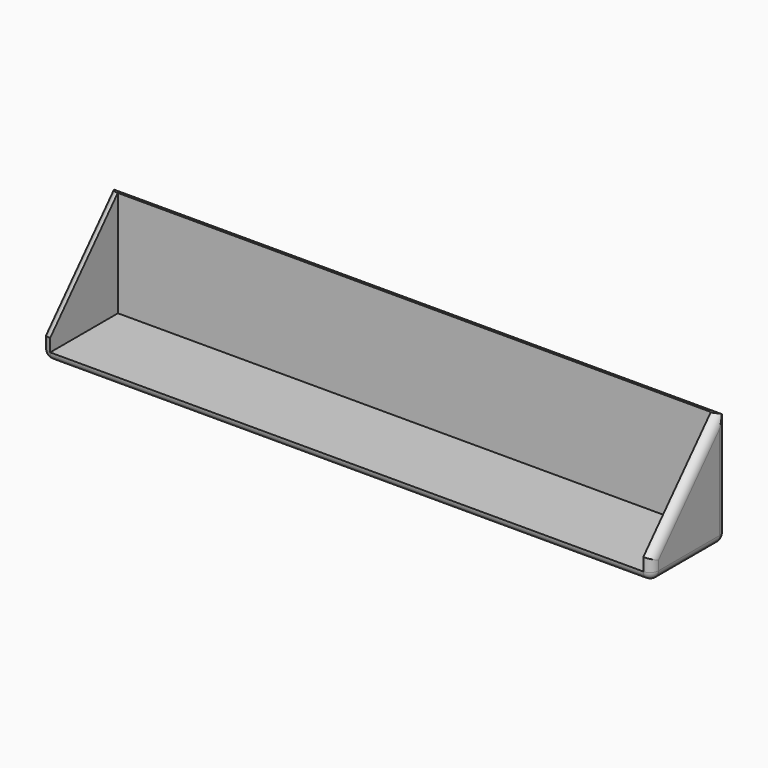
from build123d import *

# Parameters (mm, degrees)
F0_W         = 144
F0_H         = 22
F1_DEPTH     = 2
F3_DEPTH     = 25
F5_DEPTH     = 160
F6_T1_DEPTH  = 18
F6_T3_DEPTH  = 140
F6_T5_DEPTH  = 30
F6_T7_DEPTH  = 39.6649624979
F6_T9_DEPTH  = 8
F6_T11_DEPTH = 154
F6_S15_W     = 2
F6_S15_H     = 2
F6_T16_DEPTH = 2
F6_S21_W     = 2
F6_S21_H     = 2
F6_T22_DEPTH = 2
F6_S27_W     = 2
F6_S27_H     = 2
F6_T28_DEPTH = 2
F6_S33_W     = 2
F6_S33_H     = 2
F6_T34_DEPTH = 2


# Not quite as in the source:
# - a fillet or chamfer that OpenCascade refuses, or shapes differently, is made with other operations: its cross-section is extruded or revolved along the edge and cut away or added


with BuildPart() as f1:
    # F0 (on Top) → F1 (new body)
    with BuildSketch(Plane.XY):
        Rectangle(F0_W, F0_H)
    extrude(amount=F1_DEPTH)

    # F2 (on face) → F3 (join)
    with BuildSketch(Plane.XY.offset(2)):
        Polygon((-70.000000298, -11), (-70.000000298, 9.000000298), (70.000000298, 9.000000298), (70.000000298, -11), (72, -11), (72, 11), (-72, 11), (-72, -11), align=None)
    extrude(amount=F3_DEPTH)

    # F4 (on face) → F5 (cut)
    with BuildSketch(Plane(origin=(-72, 0, 0), x_dir=(0, -1, 0), z_dir=(-1, 0, 0))):
        Polygon((11, 27), (-8.9, 27), (11, 5), align=None)
    extrude(amount=-F5_DEPTH, mode=Mode.SUBTRACT)

    # F6: fillet of radius 2 on 11 edges, made by hand

    # F6_s2 → F6_t1 (cut)
    with BuildSketch(Plane.XZ.offset(-9)):
        with BuildLine():
            ThreePointArc((72, 2), (71.4142135624, 0.5857864376), (70, 0))
            Line((70, 0), (72, 0))
            Line((72, 0), (72, 2))
        make_face()
        with BuildLine():
            ThreePointArc((-70, 0), (-71.4142135624, 0.5857864376), (-72, 2))
            Line((-72, 2), (-72, 0))
            Line((-72, 0), (-70, 0))
        make_face()
    extrude(amount=F6_T1_DEPTH, mode=Mode.SUBTRACT)

    # F6_s4 → F6_t3 (cut)
    with BuildSketch(Plane.YZ.offset(-70)):
        with BuildLine():
            ThreePointArc((9, 0), (10.4142135624, 0.5857864376), (11, 2))
            Line((11, 2), (11, 0))
            Line((11, 0), (9, 0))
        make_face()
        with BuildLine():
            ThreePointArc((-11, 2), (-10.4142135624, 0.5857864376), (-9, 0))
            Line((-9, 0), (-11, 0))
            Line((-11, 0), (-11, 2))
        make_face()
    extrude(amount=F6_T3_DEPTH, mode=Mode.SUBTRACT)

    # F6_s6 → F6_t5 (cut)
    with BuildSketch(Plane.XY.offset(2)):
        with BuildLine():
            ThreePointArc((-70, 11), (-71.4142135624, 10.4142135624), (-72, 9))
            Line((-72, 9), (-72, 11))
            Line((-72, 11), (-70, 11))
        make_face()
        with BuildLine():
            ThreePointArc((72, 9), (71.4142135624, 10.4142135624), (70, 11))
            Line((70, 11), (72, 11))
            Line((72, 11), (72, 9))
        make_face()
    extrude(amount=F6_T5_DEPTH, mode=Mode.SUBTRACT)

    # F6_s8 → F6_t7 (cut)
    with BuildSketch(Plane(origin=(0, 20.7915282423, 22.9856091121), x_dir=(1, 0, 0), z_dir=(0, -0.6708250517, -0.741615635))):
        with BuildLine():
            ThreePointArc((72, 9.5118972432), (71.4142135624, 10.9261108056), (70, 11.5118972432))
            Line((70, 11.5118972432), (72, 11.5118972432))
            Line((72, 11.5118972432), (72, 9.5118972432))
        make_face()
        with BuildLine():
            ThreePointArc((-72, 9.5118972432), (-71.4142135624, 10.9261108056), (-70, 11.5118972432))
            Line((-70, 11.5118972432), (-72, 11.5118972432))
            Line((-72, 11.5118972432), (-72, 9.5118972432))
        make_face()
    extrude(amount=F6_T7_DEPTH, mode=Mode.SUBTRACT)

    # F6_s10 → F6_t9 (cut)
    with BuildSketch(Plane.XY.offset(2)):
        with BuildLine():
            ThreePointArc((-70, -11), (-71.4142135624, -10.4142135624), (-72, -9))
            Line((-72, -9), (-72, -11))
            Line((-72, -11), (-70, -11))
        make_face()
        with BuildLine():
            ThreePointArc((72, -9), (71.4142135624, -10.4142135624), (70, -11))
            Line((70, -11), (72, -11))
            Line((72, -11), (72, -9))
        make_face()
    extrude(amount=F6_T9_DEPTH, mode=Mode.SUBTRACT)

    # F6_s12 → F6_t11 (cut)
    with BuildSketch(Plane.YZ.offset(-77)):
        with BuildLine():
            ThreePointArc((11, 25), (10.4142135624, 26.4142135624), (9, 27))
            Line((9, 27), (11, 27))
            Line((11, 27), (11, 25))
        make_face()
    extrude(amount=F6_T11_DEPTH, mode=Mode.SUBTRACT)


with BuildPart() as f6_tool14:
    # F6_s15 → F6_t16 (new body)
    with BuildSketch(Plane.YZ.offset(70)):
        with Locations((-10, 1)):
            Rectangle(F6_S15_W, F6_S15_H)
    extrude(amount=F6_T16_DEPTH)

    # F6_s17 → F6_t18 (revolve, cut)
    with BuildSketch(Plane(origin=(70, -9, 2), x_dir=(0, 0.7071067812, 0.7071067812), z_dir=(0, 0.7071067812, -0.7071067812))):
        with BuildLine():
            ThreePointArc((0, -2), (2, 0), (0, 2))
            Line((0, 2), (0, -2))
        make_face()
    revolve(axis=Axis((70, -9, 2), (1, 0, 0)), mode=Mode.SUBTRACT)


with BuildPart() as f1_1:
    add(f1.part)

    # F6_t13: cut F6_tool14
    add(f6_tool14.part, mode=Mode.SUBTRACT)


with BuildPart() as f6_tool20:
    # F6_s21 → F6_t22 (new body)
    with BuildSketch(Plane.YZ.offset(70)):
        with Locations((10, 1)):
            Rectangle(F6_S21_W, F6_S21_H)
    extrude(amount=F6_T22_DEPTH)

    # F6_s23 → F6_t24 (revolve, cut)
    with BuildSketch(Plane(origin=(70, 9, 2), x_dir=(0, -0.7071067812, 0.7071067812), z_dir=(0, 0.7071067812, 0.7071067812))):
        with BuildLine():
            ThreePointArc((0, -2), (2, 0), (0, 2))
            Line((0, 2), (0, -2))
        make_face()
    revolve(axis=Axis((70, 9, 2), (1, 0, 0)), mode=Mode.SUBTRACT)


with BuildPart() as f1_2:
    add(f1_1.part)

    # F6_t19: cut F6_tool20
    add(f6_tool20.part, mode=Mode.SUBTRACT)


with BuildPart() as f6_tool26:
    # F6_s27 → F6_t28 (new body)
    with BuildSketch(Plane.XY.offset(2)):
        with Locations((-71, 10)):
            Rectangle(F6_S27_W, F6_S27_H)
    extrude(amount=-F6_T28_DEPTH)

    # F6_s29 → F6_t30 (revolve, cut)
    with BuildSketch(Plane(origin=(-70, 9, 2), x_dir=(0.7071067812, -0.7071067812, 0), z_dir=(0.7071067812, 0.7071067812, 0))):
        with BuildLine():
            ThreePointArc((0, -2), (2, 0), (0, 2))
            Line((0, 2), (0, -2))
        make_face()
    revolve(axis=Axis((-70, 9, 2), (0, 0, -1)), mode=Mode.SUBTRACT)


with BuildPart() as f1_3:
    add(f1_2.part)

    # F6_t25: cut F6_tool26
    add(f6_tool26.part, mode=Mode.SUBTRACT)


with BuildPart() as f6_tool32:
    # F6_s33 → F6_t34 (new body)
    with BuildSketch(Plane.XZ.offset(9)):
        with Locations((-71, 1)):
            Rectangle(F6_S33_W, F6_S33_H)
    extrude(amount=F6_T34_DEPTH)

    # F6_s35 → F6_t36 (revolve, cut)
    with BuildSketch(Plane(origin=(-70, -9, 2), x_dir=(0.7071067812, 0, 0.7071067812), z_dir=(0.7071067812, 0, -0.7071067812))):
        with BuildLine():
            ThreePointArc((0, -2), (2, 0), (0, 2))
            Line((0, 2), (0, -2))
        make_face()
    revolve(axis=Axis((-70, -9, 2), (0, -1, 0)), mode=Mode.SUBTRACT)


with BuildPart() as f1_4:
    add(f1_3.part)

    # F6_t31: cut F6_tool32
    add(f6_tool32.part, mode=Mode.SUBTRACT)


solid = f1_4.part
